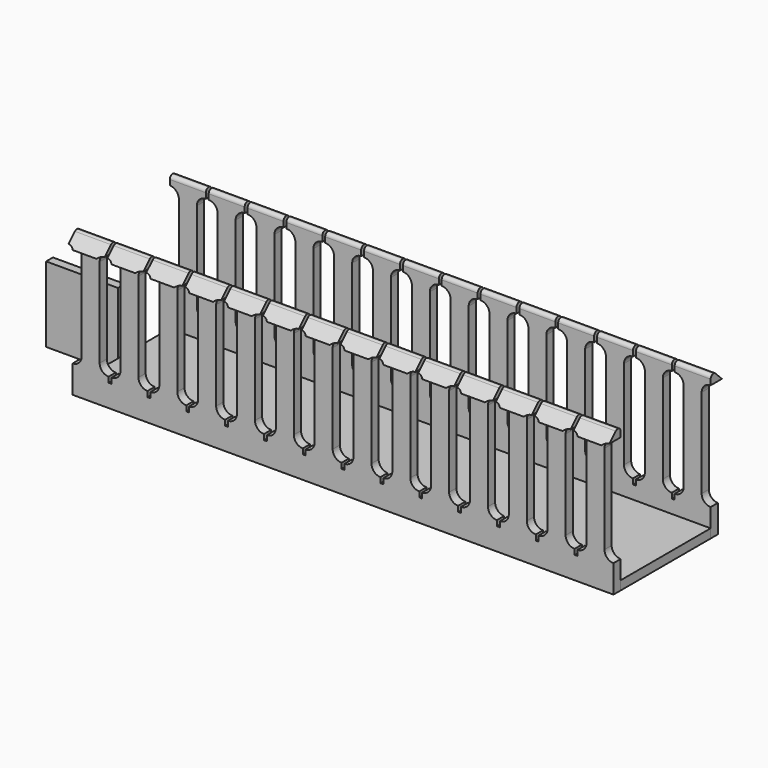
from build123d import *

# Parameters (mm, degrees)
F1_DEPTH  = 3.175
F3_DEPTH  = 191.009
F4_DEPTH  = 191.009
F6_DEPTH  = 191.008
F7_R      = 3.175
F8_DEPTH  = 2.6426
F9_W      = 1.016
F9_H      = 1.7960512242
F10_DEPTH = 25.4
F11_W     = 3.0276849866
F11_H     = 26.5962514095
F12_DEPTH = 25.4
F14_W     = 39.7309549153
F14_H     = 3.175
F15_DEPTH = 191.008


# Not quite as in the source:
# - after a boolean that leaves OpenCascade's solid faulty, fix() repairs it
# - a feature of the source that left no trace in its solid (it failed there, or was rolled back) is left out


with BuildPart() as f1:
    # F0 (on Front) → F1 (new body)
    with BuildSketch(Plane.XZ):
        with BuildLine():
            Line((0, 50.8), (0, 47.625))
            ThreePointArc((0, 47.625), (2.2450640303, 46.6950640303), (3.175, 44.45))
            Line((3.175, 44.45), (3.175, 12.954))
            ThreePointArc((3.175, 12.954), (2.2450640303, 10.7089359697), (0, 9.779))
            Line((0, 9.779), (0, 0))
            Line((0, 0), (191.008, 0))
            Line((191.008, 0), (191.008, 9.779))
            ThreePointArc((191.008, 9.779), (188.7629359697, 10.7089359697), (187.833, 12.954))
            Line((187.833, 12.954), (187.833, 44.45))
            ThreePointArc((187.833, 44.45), (188.7629359697, 46.6950640303), (191.008, 47.625))
            Line((191.008, 47.625), (191.008, 50.8))
            Line((191.008, 50.8), (178.308, 50.8))
            Line((178.308, 50.8), (178.308, 47.625))
            ThreePointArc((178.308, 47.625), (180.5530640303, 46.6950640303), (181.483, 44.45))
            Line((181.483, 44.45), (181.483, 12.954))
            ThreePointArc((181.483, 12.954), (180.5530640303, 10.7089359697), (178.308, 9.779))
            Line((178.308, 9.779), (178.308, 7.874))
            Line((178.308, 7.874), (177.292, 7.874))
            Line((177.292, 7.874), (177.292, 9.779))
            ThreePointArc((177.292, 9.779), (175.0469359697, 10.7089359697), (174.117, 12.954))
            Line((174.117, 12.954), (174.117, 44.45))
            ThreePointArc((174.117, 44.45), (175.0469359697, 46.6950640303), (177.292, 47.625))
            Line((177.292, 47.625), (177.292, 50.8))
            Line((177.292, 50.8), (164.592, 50.8))
            Line((164.592, 50.8), (164.592, 47.625))
            ThreePointArc((164.592, 47.625), (166.8370640303, 46.6950640303), (167.767, 44.45))
            Line((167.767, 44.45), (167.767, 12.954))
            ThreePointArc((167.767, 12.954), (166.8370640303, 10.7089359697), (164.592, 9.779))
            Line((164.592, 9.779), (164.592, 7.874))
            Line((164.592, 7.874), (163.576, 7.874))
            Line((163.576, 7.874), (163.576, 9.779))
            ThreePointArc((163.576, 9.779), (161.3309359697, 10.7089359697), (160.401, 12.954))
            Line((160.401, 12.954), (160.401, 44.45))
            ThreePointArc((160.401, 44.45), (161.3309359697, 46.6950640303), (163.576, 47.625))
            Line((163.576, 47.625), (163.576, 50.8))
            Line((163.576, 50.8), (150.876, 50.8))
            Line((150.876, 50.8), (150.876, 47.625))
            ThreePointArc((150.876, 47.625), (153.1210640303, 46.6950640303), (154.051, 44.45))
            Line((154.051, 44.45), (154.051, 12.954))
            ThreePointArc((154.051, 12.954), (153.1210640303, 10.7089359697), (150.876, 9.779))
            Line((150.876, 9.779), (150.876, 7.874))
            Line((150.876, 7.874), (149.86, 7.874))
            Line((149.86, 7.874), (149.86, 9.779))
            ThreePointArc((149.86, 9.779), (147.6149359697, 10.7089359697), (146.685, 12.954))
            Line((146.685, 12.954), (146.685, 44.45))
            ThreePointArc((146.685, 44.45), (147.6149359697, 46.6950640303), (149.86, 47.625))
            Line((149.86, 47.625), (149.86, 50.8))
            Line((149.86, 50.8), (137.16, 50.8))
            Line((137.16, 50.8), (137.16, 47.625))
            ThreePointArc((137.16, 47.625), (139.4050640303, 46.6950640303), (140.335, 44.45))
            Line((140.335, 44.45), (140.335, 12.954))
            ThreePointArc((140.335, 12.954), (139.4050640303, 10.7089359697), (137.16, 9.779))
            Line((137.16, 9.779), (137.16, 7.874))
            Line((137.16, 7.874), (136.144, 7.874))
            Line((136.144, 7.874), (136.144, 9.779))
            ThreePointArc((136.144, 9.779), (133.8989359697, 10.7089359697), (132.969, 12.954))
            Line((132.969, 12.954), (132.969, 44.45))
            ThreePointArc((132.969, 44.45), (133.8989359697, 46.6950640303), (136.144, 47.625))
            Line((136.144, 47.625), (136.144, 50.8))
            Line((136.144, 50.8), (123.444, 50.8))
            Line((123.444, 50.8), (123.444, 47.625))
            ThreePointArc((123.444, 47.625), (125.6890640303, 46.6950640303), (126.619, 44.45))
            Line((126.619, 44.45), (126.619, 12.954))
            ThreePointArc((126.619, 12.954), (125.6890640303, 10.7089359697), (123.444, 9.779))
            Line((123.444, 9.779), (123.444, 7.874))
            Line((123.444, 7.874), (122.428, 7.874))
            Line((122.428, 7.874), (122.428, 9.779))
            ThreePointArc((122.428, 9.779), (120.1829359697, 10.7089359697), (119.253, 12.954))
            Line((119.253, 12.954), (119.253, 44.45))
            ThreePointArc((119.253, 44.45), (120.1829359697, 46.6950640303), (122.428, 47.625))
            Line((122.428, 47.625), (122.428, 50.8))
            Line((122.428, 50.8), (109.728, 50.8))
            Line((109.728, 50.8), (109.728, 47.625))
            ThreePointArc((109.728, 47.625), (111.9730640303, 46.6950640303), (112.903, 44.45))
            Line((112.903, 44.45), (112.903, 12.954))
            ThreePointArc((112.903, 12.954), (111.9730640303, 10.7089359697), (109.728, 9.779))
            Line((109.728, 9.779), (109.728, 7.874))
            Line((109.728, 7.874), (108.712, 7.874))
            Line((108.712, 7.874), (108.712, 9.779))
            ThreePointArc((108.712, 9.779), (106.4669359697, 10.7089359697), (105.537, 12.954))
            Line((105.537, 12.954), (105.537, 44.45))
            ThreePointArc((105.537, 44.45), (106.4669359697, 46.6950640303), (108.712, 47.625))
            Line((108.712, 47.625), (108.712, 50.8))
            Line((108.712, 50.8), (96.012, 50.8))
            Line((96.012, 50.8), (96.012, 47.625))
            ThreePointArc((96.012, 47.625), (98.2570640303, 46.6950640303), (99.187, 44.45))
            Line((99.187, 44.45), (99.187, 12.954))
            ThreePointArc((99.187, 12.954), (98.2570640303, 10.7089359697), (96.012, 9.779))
            Line((96.012, 9.779), (96.012, 7.874))
            Line((96.012, 7.874), (94.996, 7.874))
            Line((94.996, 7.874), (94.996, 9.779))
            ThreePointArc((94.996, 9.779), (92.7509359697, 10.7089359697), (91.821, 12.954))
            Line((91.821, 12.954), (91.821, 44.45))
            ThreePointArc((91.821, 44.45), (92.7509359697, 46.6950640303), (94.996, 47.625))
            Line((94.996, 47.625), (94.996, 50.8))
            Line((94.996, 50.8), (82.296, 50.8))
            Line((82.296, 50.8), (82.296, 47.625))
            ThreePointArc((82.296, 47.625), (84.5410640303, 46.6950640303), (85.471, 44.45))
            Line((85.471, 44.45), (85.471, 12.954))
            ThreePointArc((85.471, 12.954), (84.5410640303, 10.7089359697), (82.296, 9.779))
            Line((82.296, 9.779), (82.296, 7.874))
            Line((82.296, 7.874), (81.28, 7.874))
            Line((81.28, 7.874), (81.28, 9.779))
            ThreePointArc((81.28, 9.779), (79.0349359697, 10.7089359697), (78.105, 12.954))
            Line((78.105, 12.954), (78.105, 44.45))
            ThreePointArc((78.105, 44.45), (79.0349359697, 46.6950640303), (81.28, 47.625))
            Line((81.28, 47.625), (81.28, 50.8))
            Line((81.28, 50.8), (68.58, 50.8))
            Line((68.58, 50.8), (68.58, 47.625))
            ThreePointArc((68.58, 47.625), (70.8250640303, 46.6950640303), (71.755, 44.45))
            Line((71.755, 44.45), (71.755, 12.954))
            ThreePointArc((71.755, 12.954), (70.8250640303, 10.7089359697), (68.58, 9.779))
            Line((68.58, 9.779), (68.58, 7.874))
            Line((68.58, 7.874), (67.564, 7.874))
            Line((67.564, 7.874), (67.564, 9.779))
            ThreePointArc((67.564, 9.779), (65.3189359697, 10.7089359697), (64.389, 12.954))
            Line((64.389, 12.954), (64.389, 44.45))
            ThreePointArc((64.389, 44.45), (65.3189359697, 46.6950640303), (67.564, 47.625))
            Line((67.564, 47.625), (67.564, 50.8))
            Line((67.564, 50.8), (54.864, 50.8))
            Line((54.864, 50.8), (54.864, 47.625))
            ThreePointArc((54.864, 47.625), (57.1090640303, 46.6950640303), (58.039, 44.45))
            Line((58.039, 44.45), (58.039, 12.954))
            ThreePointArc((58.039, 12.954), (57.1090640303, 10.7089359697), (54.864, 9.779))
            Line((54.864, 9.779), (54.864, 7.874))
            Line((54.864, 7.874), (53.848, 7.874))
            Line((53.848, 7.874), (53.848, 9.779))
            ThreePointArc((53.848, 9.779), (51.6029359697, 10.7089359697), (50.673, 12.954))
            Line((50.673, 12.954), (50.673, 44.45))
            ThreePointArc((50.673, 44.45), (51.6029359697, 46.6950640303), (53.848, 47.625))
            Line((53.848, 47.625), (53.848, 50.8))
            Line((53.848, 50.8), (41.148, 50.8))
            Line((41.148, 50.8), (41.148, 47.625))
            ThreePointArc((41.148, 47.625), (43.3930640303, 46.6950640303), (44.323, 44.45))
            Line((44.323, 44.45), (44.323, 12.954))
            ThreePointArc((44.323, 12.954), (43.3930640303, 10.7089359697), (41.148, 9.779))
            Line((41.148, 9.779), (41.148, 7.874))
            Line((41.148, 7.874), (40.132, 7.874))
            Line((40.132, 7.874), (40.132, 9.779))
            ThreePointArc((40.132, 9.779), (37.8869359697, 10.7089359697), (36.957, 12.954))
            Line((36.957, 12.954), (36.957, 44.45))
            ThreePointArc((36.957, 44.45), (37.8869359697, 46.6950640303), (40.132, 47.625))
            Line((40.132, 47.625), (40.132, 50.8))
            Line((40.132, 50.8), (27.432, 50.8))
            Line((27.432, 50.8), (27.432, 47.625))
            ThreePointArc((27.432, 47.625), (29.6770640303, 46.6950640303), (30.607, 44.45))
            Line((30.607, 44.45), (30.607, 12.954))
            ThreePointArc((30.607, 12.954), (29.6770640303, 10.7089359697), (27.432, 9.779))
            Line((27.432, 9.779), (27.432, 7.874))
            Line((27.432, 7.874), (26.416, 7.874))
            Line((26.416, 7.874), (26.416, 9.779))
            ThreePointArc((26.416, 9.779), (24.1709359697, 10.7089359697), (23.241, 12.954))
            Line((23.241, 12.954), (23.241, 44.45))
            ThreePointArc((23.241, 44.45), (24.1709359697, 46.6950640303), (26.416, 47.625))
            Line((26.416, 47.625), (26.416, 50.8))
            Line((26.416, 50.8), (13.716, 50.8))
            Line((13.716, 50.8), (13.716, 47.625))
            ThreePointArc((13.716, 47.625), (15.9610640303, 46.6950640303), (16.891, 44.45))
            Line((16.891, 44.45), (16.891, 12.954))
            ThreePointArc((16.891, 12.954), (15.9610640303, 10.7089359697), (13.716, 9.779))
            Line((13.716, 9.779), (13.716, 7.874))
            Line((13.716, 7.874), (12.7, 7.874))
            Line((12.7, 7.874), (12.7, 9.779))
            ThreePointArc((12.7, 9.779), (10.4549359697, 10.7089359697), (9.525, 12.954))
            Line((9.525, 12.954), (9.525, 44.45))
            ThreePointArc((9.525, 44.45), (10.4549359697, 46.6950640303), (12.7, 47.625))
            Line((12.7, 47.625), (12.7, 50.8))
            Line((12.7, 50.8), (0, 50.8))
        make_face()
    extrude(amount=F1_DEPTH)

    # F2 (on face) → F3 (cut, through all)
    with BuildSketch(Plane(origin=(0, 0, 0), x_dir=(0, -1, 0), z_dir=(-1, 0, 0))):
        with BuildLine():
            Line((1.27, 50.8), (0, 50.8))
            Line((0, 50.8), (0, 49.53))
            ThreePointArc((0, 49.53), (0.3719743879, 50.4280256121), (1.27, 50.8))
        make_face()
        with BuildLine():
            Line((3.175, 50.8), (1.27, 50.8))
            ThreePointArc((1.27, 50.8), (1.7560079591, 50.7033270063), (2.1680256121, 50.4280256121))
            Line((2.1680256121, 50.4280256121), (3.175, 49.4210512242))
            Line((3.175, 49.4210512242), (3.175, 50.8))
        make_face()
    extrude(amount=-F3_DEPTH, mode=Mode.SUBTRACT)

    # F2 (on face) → F4 (cut, through all)
    with BuildSketch(Plane(origin=(0, 0, 0), x_dir=(0, -1, 0), z_dir=(-1, 0, 0))):
        with BuildLine():
            Line((1.27, 50.8), (0, 50.8))
            Line((0, 50.8), (0, 49.53))
            ThreePointArc((0, 49.53), (0.3719743879, 50.4280256121), (1.27, 50.8))
        make_face()
        with BuildLine():
            Line((3.175, 50.8), (1.27, 50.8))
            ThreePointArc((1.27, 50.8), (1.7560079591, 50.7033270063), (2.1680256121, 50.4280256121))
            Line((2.1680256121, 50.4280256121), (3.175, 49.4210512242))
            Line((3.175, 49.4210512242), (3.175, 50.8))
        make_face()
    extrude(amount=-F4_DEPTH, mode=Mode.SUBTRACT)

    # F5 (on face) → F6 (join)
    with BuildSketch(Plane(origin=(0, 0, 0), x_dir=(0, -1, 0), z_dir=(-1, 0, 0))):
        Polygon((5.8166, 46.7794512242), (3.175, 49.4210512242), (3.175, 46.7794512242), align=None)
    extrude(amount=-F6_DEPTH)

    # F7 (on face) → F8 (cut, through all)
    with BuildSketch(Plane.XZ.offset(3.175)):
        with Locations((0, 44.45)):
            Circle(F7_R)
        with BuildLine():
            ThreePointArc((13.208, 41.3159034795), (15.1180079611, 42.3923648283), (15.875, 44.45))
            ThreePointArc((15.875, 44.45), (15.2857505318, 46.2924220981), (13.7367201969, 47.4509725479))
            ThreePointArc((13.7367201969, 47.4509725479), (13.4752229484, 47.5289047371), (13.208, 47.5840965205))
            ThreePointArc((13.208, 47.5840965205), (10.541, 44.45), (13.208, 41.3159034795))
        make_face()
        with BuildLine():
            ThreePointArc((13.7367201969, 47.4509725479), (15.2857505318, 46.2924220981), (15.875, 44.45))
            ThreePointArc((15.875, 44.45), (15.1180079611, 42.3923648283), (13.208, 41.3159034795))
            ThreePointArc((13.208, 41.3159034795), (15.7736351717, 42.0319920389), (16.891, 44.45))
            ThreePointArc((16.891, 44.45), (15.968377813, 46.6877263433), (13.7367201969, 47.6249323888))
            Line((13.7367201969, 47.6249323888), (13.7367201969, 47.4509725479))
        make_face()
        with BuildLine():
            ThreePointArc((13.208, 47.5840965205), (13.4752229484, 47.5289047371), (13.7367201969, 47.4509725479))
            Line((13.7367201969, 47.4509725479), (13.7367201969, 47.6249323888))
            ThreePointArc((13.7367201969, 47.6249323888), (13.4715060458, 47.6155722557), (13.208, 47.5840965205))
        make_face()
        with BuildLine():
            ThreePointArc((13.208, 47.5840965205), (9.525, 44.45), (13.208, 41.3159034795))
            ThreePointArc((13.208, 41.3159034795), (10.541, 44.45), (13.208, 47.5840965205))
        make_face()
        with BuildLine():
            ThreePointArc((26.924, 41.3159034795), (28.8340079611, 42.3923648283), (29.591, 44.45))
            ThreePointArc((29.591, 44.45), (28.8340079611, 46.5076351717), (26.924, 47.5840965205))
            ThreePointArc((26.924, 47.5840965205), (24.257, 44.45), (26.924, 41.3159034795))
        make_face()
        with BuildLine():
            ThreePointArc((26.924, 47.5840965205), (28.8340079611, 46.5076351717), (29.591, 44.45))
            ThreePointArc((29.591, 44.45), (28.8340079611, 42.3923648283), (26.924, 41.3159034795))
            ThreePointArc((26.924, 41.3159034795), (29.4896351717, 42.0319920389), (30.607, 44.45))
            ThreePointArc((30.607, 44.45), (29.4896351717, 46.8680079611), (26.924, 47.5840965205))
        make_face()
        with BuildLine():
            ThreePointArc((26.924, 41.3159034795), (24.257, 44.45), (26.924, 47.5840965205))
            ThreePointArc((26.924, 47.5840965205), (23.241, 44.45), (26.924, 41.3159034795))
        make_face()
        with BuildLine():
            ThreePointArc((40.64, 41.3159034795), (42.5500079611, 42.3923648283), (43.307, 44.45))
            ThreePointArc((43.307, 44.45), (42.5500079611, 46.5076351717), (40.64, 47.5840965205))
            ThreePointArc((40.64, 47.5840965205), (37.973, 44.45), (40.64, 41.3159034795))
        make_face()
        with BuildLine():
            ThreePointArc((40.64, 47.5840965205), (42.5500079611, 46.5076351717), (43.307, 44.45))
            ThreePointArc((43.307, 44.45), (42.5500079611, 42.3923648283), (40.64, 41.3159034795))
            ThreePointArc((40.64, 41.3159034795), (43.2056351717, 42.0319920389), (44.323, 44.45))
            ThreePointArc((44.323, 44.45), (43.2056351717, 46.8680079611), (40.64, 47.5840965205))
        make_face()
        with BuildLine():
            ThreePointArc((40.64, 41.3159034795), (37.973, 44.45), (40.64, 47.5840965205))
            ThreePointArc((40.64, 47.5840965205), (36.957, 44.45), (40.64, 41.3159034795))
        make_face()
        with BuildLine():
            ThreePointArc((54.356, 41.3159034795), (56.2660079611, 42.3923648283), (57.023, 44.45))
            ThreePointArc((57.023, 44.45), (56.2660079611, 46.5076351717), (54.356, 47.5840965205))
            ThreePointArc((54.356, 47.5840965205), (51.689, 44.45), (54.356, 41.3159034795))
        make_face()
        with BuildLine():
            ThreePointArc((54.356, 47.5840965205), (56.2660079611, 46.5076351717), (57.023, 44.45))
            ThreePointArc((57.023, 44.45), (56.2660079611, 42.3923648283), (54.356, 41.3159034795))
            ThreePointArc((54.356, 41.3159034795), (56.9216351717, 42.0319920389), (58.039, 44.45))
            ThreePointArc((58.039, 44.45), (56.9216351717, 46.8680079611), (54.356, 47.5840965205))
        make_face()
        with BuildLine():
            ThreePointArc((54.356, 41.3159034795), (51.689, 44.45), (54.356, 47.5840965205))
            ThreePointArc((54.356, 47.5840965205), (50.673, 44.45), (54.356, 41.3159034795))
        make_face()
        with BuildLine():
            ThreePointArc((68.072, 41.3159034795), (69.9820079611, 42.3923648283), (70.739, 44.45))
            ThreePointArc((70.739, 44.45), (69.9820079611, 46.5076351717), (68.072, 47.5840965205))
            ThreePointArc((68.072, 47.5840965205), (65.405, 44.45), (68.072, 41.3159034795))
        make_face()
        with BuildLine():
            ThreePointArc((68.072, 47.5840965205), (69.9820079611, 46.5076351717), (70.739, 44.45))
            ThreePointArc((70.739, 44.45), (69.9820079611, 42.3923648283), (68.072, 41.3159034795))
            ThreePointArc((68.072, 41.3159034795), (70.6376351717, 42.0319920389), (71.755, 44.45))
            ThreePointArc((71.755, 44.45), (70.6376351717, 46.8680079611), (68.072, 47.5840965205))
        make_face()
        with BuildLine():
            ThreePointArc((68.072, 41.3159034795), (65.405, 44.45), (68.072, 47.5840965205))
            ThreePointArc((68.072, 47.5840965205), (64.389, 44.45), (68.072, 41.3159034795))
        make_face()
        with BuildLine():
            ThreePointArc((81.788, 41.3159034795), (83.6980079611, 42.3923648283), (84.455, 44.45))
            ThreePointArc((84.455, 44.45), (83.6980079611, 46.5076351717), (81.788, 47.5840965205))
            ThreePointArc((81.788, 47.5840965205), (79.121, 44.45), (81.788, 41.3159034795))
        make_face()
        with BuildLine():
            ThreePointArc((81.788, 47.5840965205), (83.6980079611, 46.5076351717), (84.455, 44.45))
            ThreePointArc((84.455, 44.45), (83.6980079611, 42.3923648283), (81.788, 41.3159034795))
            ThreePointArc((81.788, 41.3159034795), (84.3536351717, 42.0319920389), (85.471, 44.45))
            ThreePointArc((85.471, 44.45), (84.3536351717, 46.8680079611), (81.788, 47.5840965205))
        make_face()
        with BuildLine():
            ThreePointArc((81.788, 41.3159034795), (79.121, 44.45), (81.788, 47.5840965205))
            ThreePointArc((81.788, 47.5840965205), (78.105, 44.45), (81.788, 41.3159034795))
        make_face()
        with BuildLine():
            ThreePointArc((95.504, 41.3159034795), (97.4140079611, 42.3923648283), (98.171, 44.45))
            ThreePointArc((98.171, 44.45), (97.4140079611, 46.5076351717), (95.504, 47.5840965205))
            ThreePointArc((95.504, 47.5840965205), (92.837, 44.45), (95.504, 41.3159034795))
        make_face()
        with BuildLine():
            ThreePointArc((95.504, 47.5840965205), (97.4140079611, 46.5076351717), (98.171, 44.45))
            ThreePointArc((98.171, 44.45), (97.4140079611, 42.3923648283), (95.504, 41.3159034795))
            ThreePointArc((95.504, 41.3159034795), (98.0696351717, 42.0319920389), (99.187, 44.45))
            ThreePointArc((99.187, 44.45), (98.0696351717, 46.8680079611), (95.504, 47.5840965205))
        make_face()
        with BuildLine():
            ThreePointArc((95.504, 41.3159034795), (92.837, 44.45), (95.504, 47.5840965205))
            ThreePointArc((95.504, 47.5840965205), (91.821, 44.45), (95.504, 41.3159034795))
        make_face()
        with BuildLine():
            ThreePointArc((109.22, 41.3159034795), (111.1300079611, 42.3923648283), (111.887, 44.45))
            ThreePointArc((111.887, 44.45), (111.1300079611, 46.5076351717), (109.22, 47.5840965205))
            ThreePointArc((109.22, 47.5840965205), (106.553, 44.45), (109.22, 41.3159034795))
        make_face()
        with BuildLine():
            ThreePointArc((109.22, 47.5840965205), (111.1300079611, 46.5076351717), (111.887, 44.45))
            ThreePointArc((111.887, 44.45), (111.1300079611, 42.3923648283), (109.22, 41.3159034795))
            ThreePointArc((109.22, 41.3159034795), (111.7856351717, 42.0319920389), (112.903, 44.45))
            ThreePointArc((112.903, 44.45), (111.7856351717, 46.8680079611), (109.22, 47.5840965205))
        make_face()
        with BuildLine():
            ThreePointArc((109.22, 41.3159034795), (106.553, 44.45), (109.22, 47.5840965205))
            ThreePointArc((109.22, 47.5840965205), (105.537, 44.45), (109.22, 41.3159034795))
        make_face()
        with BuildLine():
            ThreePointArc((122.936, 41.3159034795), (124.8460079611, 42.3923648283), (125.603, 44.45))
            ThreePointArc((125.603, 44.45), (124.8460079611, 46.5076351717), (122.936, 47.5840965205))
            ThreePointArc((122.936, 47.5840965205), (120.269, 44.45), (122.936, 41.3159034795))
        make_face()
        with BuildLine():
            ThreePointArc((122.936, 47.5840965205), (124.8460079611, 46.5076351717), (125.603, 44.45))
            ThreePointArc((125.603, 44.45), (124.8460079611, 42.3923648283), (122.936, 41.3159034795))
            ThreePointArc((122.936, 41.3159034795), (125.5016351717, 42.0319920389), (126.619, 44.45))
            ThreePointArc((126.619, 44.45), (125.5016351717, 46.8680079611), (122.936, 47.5840965205))
        make_face()
        with BuildLine():
            ThreePointArc((122.936, 41.3159034795), (120.269, 44.45), (122.936, 47.5840965205))
            ThreePointArc((122.936, 47.5840965205), (119.253, 44.45), (122.936, 41.3159034795))
        make_face()
        with BuildLine():
            ThreePointArc((136.652, 41.3159034795), (138.5620079611, 42.3923648283), (139.319, 44.45))
            ThreePointArc((139.319, 44.45), (138.5620079611, 46.5076351717), (136.652, 47.5840965205))
            ThreePointArc((136.652, 47.5840965205), (133.985, 44.45), (136.652, 41.3159034795))
        make_face()
        with BuildLine():
            ThreePointArc((136.652, 47.5840965205), (138.5620079611, 46.5076351717), (139.319, 44.45))
            ThreePointArc((139.319, 44.45), (138.5620079611, 42.3923648283), (136.652, 41.3159034795))
            ThreePointArc((136.652, 41.3159034795), (139.2176351717, 42.0319920389), (140.335, 44.45))
            ThreePointArc((140.335, 44.45), (139.2176351717, 46.8680079611), (136.652, 47.5840965205))
        make_face()
        with BuildLine():
            ThreePointArc((136.652, 41.3159034795), (133.985, 44.45), (136.652, 47.5840965205))
            ThreePointArc((136.652, 47.5840965205), (132.969, 44.45), (136.652, 41.3159034795))
        make_face()
        with BuildLine():
            ThreePointArc((150.368, 41.3159034795), (152.2780079611, 42.3923648283), (153.035, 44.45))
            ThreePointArc((153.035, 44.45), (152.2780079611, 46.5076351717), (150.368, 47.5840965205))
            ThreePointArc((150.368, 47.5840965205), (147.701, 44.45), (150.368, 41.3159034795))
        make_face()
        with BuildLine():
            ThreePointArc((150.368, 47.5840965205), (152.2780079611, 46.5076351717), (153.035, 44.45))
            ThreePointArc((153.035, 44.45), (152.2780079611, 42.3923648283), (150.368, 41.3159034795))
            ThreePointArc((150.368, 41.3159034795), (152.9336351717, 42.0319920389), (154.051, 44.45))
            ThreePointArc((154.051, 44.45), (152.9336351717, 46.8680079611), (150.368, 47.5840965205))
        make_face()
        with BuildLine():
            ThreePointArc((150.368, 41.3159034795), (147.701, 44.45), (150.368, 47.5840965205))
            ThreePointArc((150.368, 47.5840965205), (146.685, 44.45), (150.368, 41.3159034795))
        make_face()
        with BuildLine():
            ThreePointArc((164.084, 41.3159034795), (165.9940079611, 42.3923648283), (166.751, 44.45))
            ThreePointArc((166.751, 44.45), (165.9940079611, 46.5076351717), (164.084, 47.5840965205))
            ThreePointArc((164.084, 47.5840965205), (161.417, 44.45), (164.084, 41.3159034795))
        make_face()
        with BuildLine():
            ThreePointArc((164.084, 47.5840965205), (165.9940079611, 46.5076351717), (166.751, 44.45))
            ThreePointArc((166.751, 44.45), (165.9940079611, 42.3923648283), (164.084, 41.3159034795))
            ThreePointArc((164.084, 41.3159034795), (166.6496351717, 42.0319920389), (167.767, 44.45))
            ThreePointArc((167.767, 44.45), (166.6496351717, 46.8680079611), (164.084, 47.5840965205))
        make_face()
        with BuildLine():
            ThreePointArc((164.084, 41.3159034795), (161.417, 44.45), (164.084, 47.5840965205))
            ThreePointArc((164.084, 47.5840965205), (160.401, 44.45), (164.084, 41.3159034795))
        make_face()
        with BuildLine():
            ThreePointArc((177.8, 41.3159034795), (179.7100079611, 42.3923648283), (180.467, 44.45))
            ThreePointArc((180.467, 44.45), (179.7100079611, 46.5076351717), (177.8, 47.5840965205))
            ThreePointArc((177.8, 47.5840965205), (175.133, 44.45), (177.8, 41.3159034795))
        make_face()
        with BuildLine():
            ThreePointArc((177.8, 47.5840965205), (179.7100079611, 46.5076351717), (180.467, 44.45))
            ThreePointArc((180.467, 44.45), (179.7100079611, 42.3923648283), (177.8, 41.3159034795))
            ThreePointArc((177.8, 41.3159034795), (180.3656351717, 42.0319920389), (181.483, 44.45))
            ThreePointArc((181.483, 44.45), (180.3656351717, 46.8680079611), (177.8, 47.5840965205))
        make_face()
        with BuildLine():
            ThreePointArc((177.8, 41.3159034795), (175.133, 44.45), (177.8, 47.5840965205))
            ThreePointArc((177.8, 47.5840965205), (174.117, 44.45), (177.8, 41.3159034795))
        make_face()
        with Locations((191.008, 44.45)):
            Circle(F7_R)
    extrude(amount=F8_DEPTH, mode=Mode.SUBTRACT)

    add(f1.part.fix(), mode=Mode.REPLACE)

    # F9 (on face) → F10 (cut)
    with BuildSketch(Plane(origin=(0, -3.175, 0), x_dir=(-1, 0, 0), z_dir=(0, 1, 0))):
        with Locations((-13.208, 48.5230256121)):
            Rectangle(F9_W, F9_H)
        Polygon((-12.7, 47.625), (-13.716, 47.625), (-13.208, 47.5840965205), align=None)
        with Locations((-26.924, 48.5230256121)):
            Rectangle(F9_W, F9_H)
        Polygon((-26.416, 47.625), (-27.432, 47.625), (-26.924, 47.5840965205), align=None)
        with Locations((-40.64, 48.5230256121)):
            Rectangle(F9_W, F9_H)
        Polygon((-40.132, 47.625), (-41.148, 47.625), (-40.64, 47.5840965205), align=None)
        with Locations((-68.072, 48.5230256121)):
            Rectangle(F9_W, F9_H)
        Polygon((-67.564, 47.625), (-68.58, 47.625), (-68.072, 47.5840965205), align=None)
        with Locations((-81.788, 48.5230256121)):
            Rectangle(F9_W, F9_H)
        Polygon((-81.28, 47.625), (-82.296, 47.625), (-81.788, 47.5840965205), align=None)
        with Locations((-95.504, 48.5230256121)):
            Rectangle(F9_W, F9_H)
        Polygon((-94.996, 47.625), (-96.012, 47.625), (-95.504, 47.5840965205), align=None)
        with Locations((-109.22, 48.5230256121)):
            Rectangle(F9_W, F9_H)
        Polygon((-108.712, 47.625), (-109.728, 47.625), (-109.22, 47.5840965205), align=None)
        with Locations((-54.356, 48.5230256121)):
            Rectangle(F9_W, F9_H)
        Polygon((-53.848, 47.625), (-54.864, 47.625), (-54.356, 47.5840965205), align=None)
        with Locations((-122.936, 48.5230256121)):
            Rectangle(F9_W, F9_H)
        Polygon((-122.428, 47.625), (-123.444, 47.625), (-122.936, 47.5840965205), align=None)
        with Locations((-136.652, 48.5230256121)):
            Rectangle(F9_W, F9_H)
        Polygon((-136.144, 47.625), (-137.16, 47.625), (-136.652, 47.5840965205), align=None)
        with Locations((-150.368, 48.5230256121)):
            Rectangle(F9_W, F9_H)
        Polygon((-149.86, 47.625), (-150.876, 47.625), (-150.368, 47.5840965205), align=None)
        with Locations((-164.084, 48.5230256121)):
            Rectangle(F9_W, F9_H)
        Polygon((-164.084, 47.5840965205), (-163.576, 47.625), (-164.592, 47.625), align=None)
        with Locations((-177.8, 48.5230256121)):
            Rectangle(F9_W, F9_H)
        Polygon((-177.292, 47.625), (-178.308, 47.625), (-177.8, 47.5840965205), align=None)
    extrude(amount=-F10_DEPTH, mode=Mode.SUBTRACT)


with BuildPart() as f12:
    # F11 (on face) → F12 (new body)
    with BuildSketch(Plane(origin=(0, 0, 0), x_dir=(0, -1, 0), z_dir=(-1, 0, 0))):
        with Locations((-18.3515734971, 11.8016155902)):
            Rectangle(F11_W, F11_H)
    extrude(amount=F12_DEPTH)


with BuildPart() as f13_1:
    # F13: instance of F1
    add(f1.part.mirror(Plane(origin=(-12.7, 19.8654159904, 11.8016155902), x_dir=(-1, 0, 0), z_dir=(0, 1, 0))))


with BuildPart() as f15:
    # F14 (on face) → F15 (new body)
    with BuildSketch(Plane(origin=(0, 0, 0), x_dir=(0, -1, 0), z_dir=(-1, 0, 0))):
        with Locations((-19.8654774576, 1.5875)):
            Rectangle(F14_W, F14_H)
    extrude(amount=-F15_DEPTH)


solid = Compound([f1.part, f12.part, f13_1.part, f15.part])
